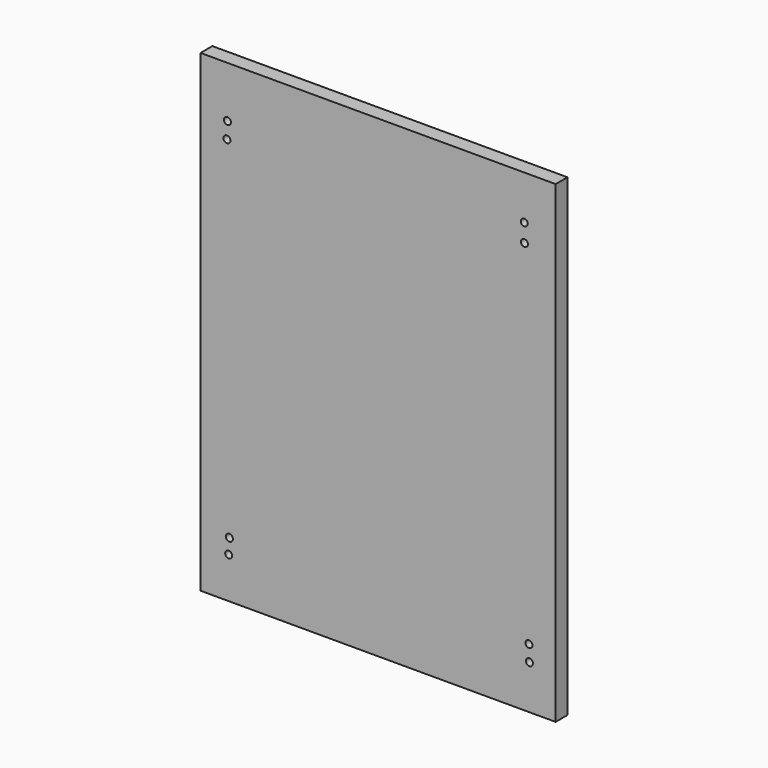
from build123d import *

# Parameters (mm, degrees)
F0_W      = 152.4
F0_H      = 203.2
F1_DEPTH  = 6.35
F3_R      = 1.5
F3_R_2    = 0.15
F6_DEPTH  = 6.35
F4_R      = 1.5
F7_DEPTH  = 6.35
F8_R      = 1.5
F9_DEPTH  = 6.35
F10_R     = 1.5
F11_DEPTH = 6.35
F12_R     = 1.5
F13_DEPTH = 6.35


# Not quite as in the source:
# - the program builds the solid bodies; features that only make, move or delete a surface that nothing else refers to are left out


with BuildPart() as f1:
    # F0 (on Front) → F1 (new body)
    with BuildSketch(Plane.XZ):
        Rectangle(F0_W, F0_H)
    extrude(amount=F1_DEPTH)

    # F3 (on face) → F6 (cut)
    with BuildSketch(Plane.XZ.offset(6.35)):
        with Locations((-64.6446496248, 79.6310603619)):
            Circle(F3_R)
        with Locations((-64.5674839616, 72.9324966669)):
            Circle(F3_R_2)
    extrude(amount=-F6_DEPTH, mode=Mode.SUBTRACT)

    # F4 (on face) → F7 (cut)
    with BuildSketch(Plane.XZ.offset(6.35)):
        with Locations((-64.8668259382, 72.6331546903)):
            Circle(F4_R)
    extrude(amount=-F7_DEPTH, mode=Mode.SUBTRACT)

    # F8 (on face) → F9 (cut)
    with BuildSketch(Plane.XZ.offset(6.35)):
        with Locations((62.737300992, 82.7085599303)):
            Circle(F8_R)
        with Locations((62.7969279885, 75.0102698803)):
            Circle(F8_R)
    extrude(amount=-F9_DEPTH, mode=Mode.SUBTRACT)

    # F10 (on face) → F11 (cut)
    with BuildSketch(Plane.XZ.offset(6.35)):
        with Locations((-63.819848001, -77.5382146239)):
            Circle(F10_R)
        with Locations((-64.1196668148, -83.984285593)):
            Circle(F10_R)
    extrude(amount=-F11_DEPTH, mode=Mode.SUBTRACT)

    # F12 (on face) → F13 (cut)
    with BuildSketch(Plane.XZ.offset(6.35)):
        with Locations((64.7413730621, -75.9207308292)):
            Circle(F12_R)
        with Locations((64.9533718824, -82.7048197389)):
            Circle(F12_R)
    extrude(amount=-F13_DEPTH, mode=Mode.SUBTRACT)


solid = f1.part
